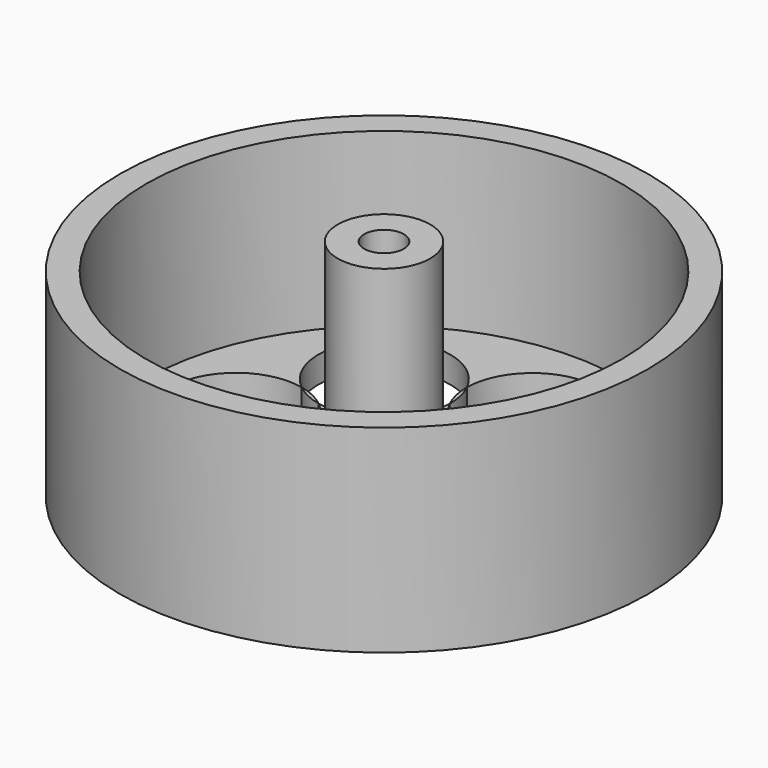
from build123d import *

# Parameters (mm, degrees)
F0_R     = 20
F1_DEPTH = 15
F2_R     = 18
F3_DEPTH = 13
F4_R     = 3.5
F4_R_2   = 1.5
F5_DEPTH = 15
F7_DEPTH = 2


# Not quite as in the source:
# - a feature names something its author has since deleted; it is built from what else it names


with BuildPart() as f1:
    # F0 (on Top) → F1 (new body)
    with BuildSketch(Plane.XY):
        Circle(F0_R)
    extrude(amount=F1_DEPTH)

    # F2 (on face) → F3 (cut)
    with BuildSketch(Plane.XY.offset(15)):
        Circle(F2_R)
    extrude(amount=-F3_DEPTH, mode=Mode.SUBTRACT)

    # F4 (on face) → F5 (join)
    with BuildSketch(Plane.XY.offset(2)):
        Circle(F4_R)
        Circle(F4_R_2, mode=Mode.SUBTRACT)
    extrude(amount=F5_DEPTH)

    # F6 (on face) → F7 (cut)
    with BuildSketch(Plane(origin=(0, 0, 0), x_dir=(1, 0, 0), z_dir=(0, 0, -1))):
        with BuildLine():
            ThreePointArc((-8.0447609019, -3.8741526647), (-6.6887361359, -2.1442685218), (-6.2056059045, 0))
            ThreePointArc((-6.2056059045, 0), (-6.6887361359, 2.1442685218), (-8.0447609019, 3.8741526647))
            ThreePointArc((-8.0447609019, 3.8741526647), (-9.1559997007, 4.2560511367), (-10.1474260077, 4.8867428115))
            ThreePointArc((-10.1474260077, 4.8867428115), (-16.2056059045, 0), (-10.1474260077, -4.8867428115))
            ThreePointArc((-10.1474260077, -4.8867428115), (-9.1559997007, -4.2560511367), (-8.0447609019, -3.8741526647))
        make_face()
        with BuildLine():
            ThreePointArc((7.0222366791, 8.8056062773), (6.4026393038, 7.8072089599), (5.5671472783, 6.9809818809))
            ThreePointArc((5.5671472783, 6.9809818809), (5.5910577264, 2.6925114933), (8.9290109664, 0))
            ThreePointArc((8.9290109664, 0), (10.0959020659, 0.1380698111), (11.2627931654, 0))
            ThreePointArc((11.2627931654, 0), (14.0223798449, 1.7663248763), (15.0959020659, 4.8619301889))
            ThreePointArc((15.0959020659, 4.8619301889), (12.2904034974, 9.3546090632), (7.0222366791, 8.8056062773))
        make_face()
        with BuildLine():
            ThreePointArc((8.9290109664, 0), (5.5910577264, -2.6925114933), (5.5671472783, -6.9809818809))
            ThreePointArc((5.5671472783, -6.9809818809), (6.4026393038, -7.8072089599), (7.0222366791, -8.8056062773))
            ThreePointArc((7.0222366791, -8.8056062773), (12.2904034974, -9.3546090632), (15.0959020659, -4.8619301889))
            ThreePointArc((15.0959020659, -4.8619301889), (14.0223798449, -1.7663248763), (11.2627931654, 0))
            ThreePointArc((11.2627931654, 0), (10.0959020659, -0.1380698111), (8.9290109664, 0))
        make_face()
        with BuildLine():
            ThreePointArc((5.5671472783, -6.9809818809), (1.3808772216, -6.0500184083), (-1.9868918596, -8.7051420193))
            ThreePointArc((-1.9868918596, -8.7051420193), (-1.9866587193, -8.7330183145), (-1.9865810051, -8.7608954763))
            ThreePointArc((-1.9865810051, -8.7608954763), (-2.118220462, -9.9006610761), (-2.5062072541, -10.9804114261))
            ThreePointArc((-2.5062072541, -10.9804114261), (2.5213590532, -15.924580255), (7.4934818914, -10.9246579692))
            ThreePointArc((7.4934818914, -10.9246579692), (7.3742489386, -9.8392488156), (7.0222366791, -8.8056062773))
            ThreePointArc((7.0222366791, -8.8056062773), (6.1867446536, -7.9793791982), (5.5671472783, -6.9809818809))
        make_face()
        with BuildLine():
            ThreePointArc((-1.9868918596, -8.7051420193), (-3.8691319958, -4.8517380639), (-8.0447609019, -3.8741526647))
            ThreePointArc((-8.0447609019, -3.8741526647), (-9.0361872089, -4.5048443395), (-10.1474260077, -4.8867428115))
            ThreePointArc((-10.1474260077, -4.8867428115), (-10.1040300144, -12.6700528886), (-2.5062072541, -10.9804114261))
            ThreePointArc((-2.5062072541, -10.9804114261), (-2.3811576695, -9.8120532994), (-1.9868918596, -8.7051420193))
        make_face()
    extrude(amount=-F7_DEPTH, mode=Mode.SUBTRACT)


solid = f1.part
